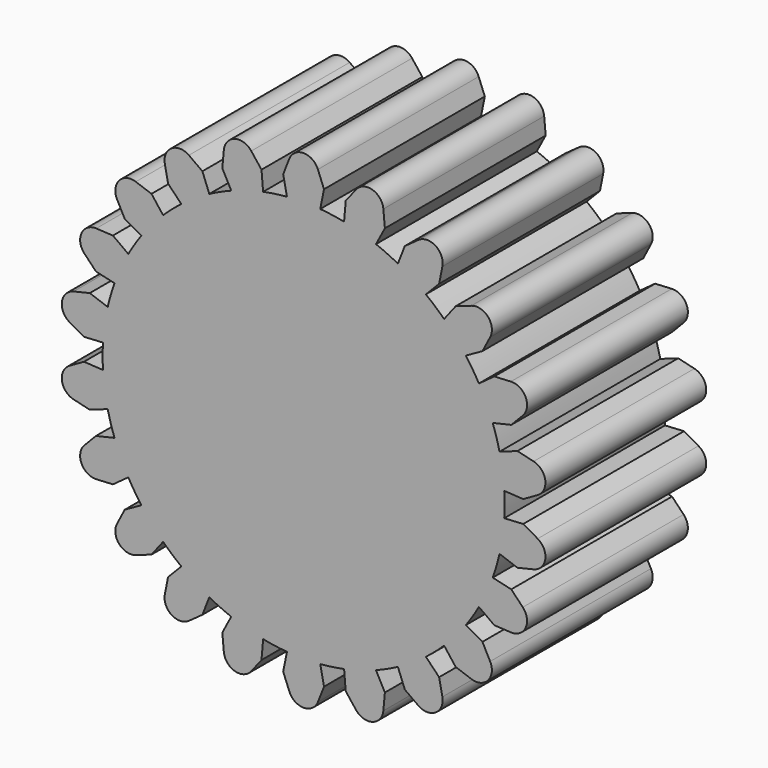
from build123d import *

# Parameters (mm, degrees)
F0_R             = 25.4
F1_DEPTH         = 25.4
F4_DEPTH         = 25.4
F4_COPIES_COUNT  = 8
F4_COPIES_ANGLE  = 343.6356
F4_COPIES1_COUNT = 3
F4_COPIES1_ANGLE = 32.7272727273
F4_COPIES2_COUNT = 3
F4_COPIES2_ANGLE = 130.9088
F4_COPIES3_COUNT = 3
F4_COPIES3_ANGLE = 163.636
F4_COPIES4_COUNT = 3
F4_COPIES4_ANGLE = 229.0904


# Not quite as in the source:
# - a pattern or mirror of a feature is missing from the dataset's text; its kind, count and spacing are read off the source's solid


with BuildPart() as f1:
    # F0 (on Front) → F1 (new body)
    with BuildSketch(Plane.XZ):
        Circle(F0_R)
    extrude(amount=F1_DEPTH)

    # F3 (on Front) → F4 (join)
    with BuildSketch(Plane.XZ):
        with BuildLine():
            ThreePointArc((-2.0394499691, 25.0140055699), (0, 25.0970084039), (2.0394499691, 25.0140055699))
            Line((2.0394499691, 25.0140055699), (2.5789397816, 27.6699554159))
            Line((2.5789397816, 27.6699554159), (1.8071979284, 29.6250353105))
            ThreePointArc((1.8071979284, 29.6250353105), (0, 30.8545671303), (-1.8071979284, 29.6250353105))
            Line((-1.8071979284, 29.6250353105), (-2.5789397816, 27.6699554159))
            Line((-2.5789397816, 27.6699554159), (-2.0394499691, 25.0140055699))
        make_face()
    f4 = extrude(amount=F4_DEPTH)

    # F4_copies: F4 ×8 about axis
    f4_copies_axis = Axis((0, 0, 0), (0, -1, 0))
    for i in range(1, F4_COPIES_COUNT):
        add(f4.rotate(f4_copies_axis, i * F4_COPIES_ANGLE / (F4_COPIES_COUNT - 1)))

    # F4_copies1: F4 ×3 about axis
    f4_copies1_axis = Axis((0, 0, 0), (0, -1, 0))
    for i in range(1, F4_COPIES1_COUNT):
        add(f4.rotate(f4_copies1_axis, i * F4_COPIES1_ANGLE / (F4_COPIES1_COUNT - 1)))

    # F4_copies2: F4 ×3 about axis
    f4_copies2_axis = Axis((0, 0, 0), (0, -1, 0))
    for i in range(1, F4_COPIES2_COUNT):
        add(f4.rotate(f4_copies2_axis, i * F4_COPIES2_ANGLE / (F4_COPIES2_COUNT - 1)))

    # F4_copies3: F4 ×3 about axis
    f4_copies3_axis = Axis((0, 0, 0), (0, -1, 0))
    for i in range(1, F4_COPIES3_COUNT):
        add(f4.rotate(f4_copies3_axis, i * F4_COPIES3_ANGLE / (F4_COPIES3_COUNT - 1)))

    # F4_copies4: F4 ×3 about axis
    f4_copies4_axis = Axis((0, 0, 0), (0, -1, 0))
    for i in range(1, F4_COPIES4_COUNT):
        add(f4.rotate(f4_copies4_axis, i * F4_COPIES4_ANGLE / (F4_COPIES4_COUNT - 1)))

    # F4_copies5: F4 across plane
    add(f4.mirror(Plane(origin=(0, 0, 0), x_dir=(-0.7557528993, 0, -0.6548568968), z_dir=(0.6548568968, 0, -0.7557528993))))

    # F4_copies6: F4 across plane
    add(f4.mirror(Plane(origin=(0, 0, 0), x_dir=(-0.9594941358, 0, -0.2817285986), z_dir=(0.2817285986, 0, -0.9594941358))))

    # F4_copies7: F4 across plane
    add(f4.mirror(Plane(origin=(0, 0, 0), x_dir=(-1, 0, 1e-06), z_dir=(-1e-06, 0, -1))))

    # F4_copies8: F4 across plane
    add(f4.mirror(Plane(origin=(0, 0, 0), x_dir=(0.4154204975, 0, 0.9096294907), z_dir=(0.9096294907, 0, -0.4154204975))))

    # F4_copies9: F4 across plane
    add(f4.mirror(Plane(origin=(0, 0, 0), x_dir=(0.6548648109, 0, 0.7557460416), z_dir=(0.7557460416, 0, -0.6548648109))))

    # F4_copies10: F4 across plane
    add(f4.mirror(Plane(origin=(0, 0, 0), x_dir=(0.2817386464, 0, 0.9594911855), z_dir=(0.9594911855, 0, -0.2817386464))))


solid = f1.part
